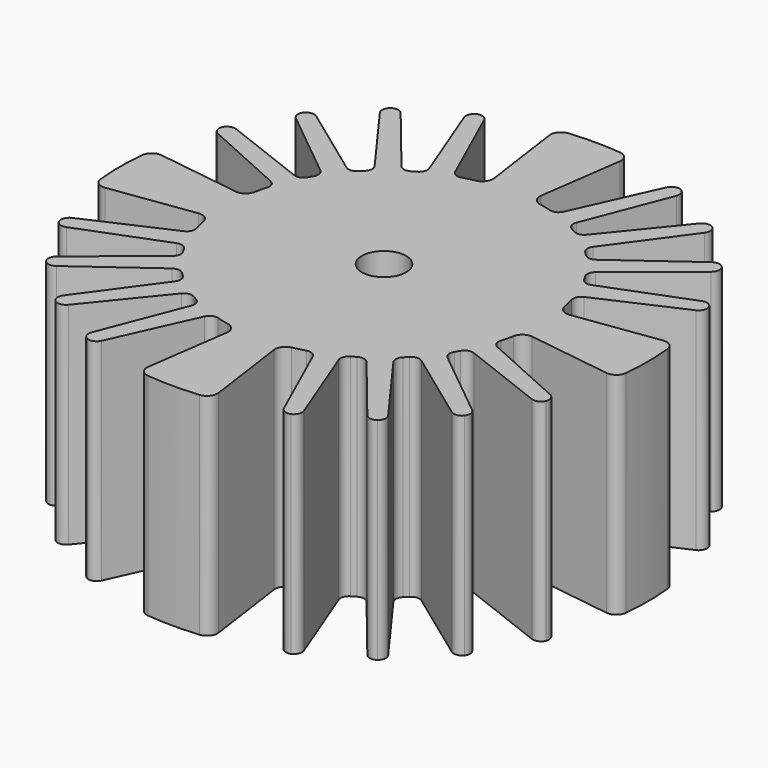
from build123d import *

# Parameters (mm, degrees)
F1_DEPTH        = 20
F2_DEPTH        = 20
F3_R            = 1
F4_DEPTH        = 20
F4_COPIES_COUNT = 4
F4_COPIES_ANGLE = 44.6001
F5_T1_DEPTH     = 20
F5_T3_DEPTH     = 23.9033983658
F6_COUNT        = 4


# Not quite as in the source:
# - a fillet or chamfer that OpenCascade refuses, or shapes differently, is made with other operations: its cross-section is extruded or revolved along the edge and cut away or added
# - a pattern or mirror of a feature is missing from the dataset's text; its kind, count and spacing are read off the source's solid


with BuildPart() as f1:
    # F0 (on Top) → F1 (new body)
    with BuildSketch(Plane.XY):
        with BuildLine():
            ThreePointArc((15, 0), (12.7601203075, 7.8853871013), (6.7094227017, 13.4157984112))
            ThreePointArc((6.7094227017, 13.4157984112), (5.7885906349, 13.8380713418), (4.8413562627, 14.19722753))
            ThreePointArc((4.8413562627, 14.19722753), (3.4800059012, 14.5907353799), (2.0875965144, 14.8540210311))
            ThreePointArc((2.0875965144, 14.8540210311), (0, 15), (-2.0875965144, 14.8540210311))
            ThreePointArc((-2.0875965144, 14.8540210311), (-9.8408854349, -11.3206437033), (15, 0))
        make_face()
    extrude(amount=F1_DEPTH)

    # F0 (on Top) → F2 (join, through all)
    with BuildSketch(Plane.XY):
        with BuildLine():
            ThreePointArc((3.479327524, 24.7567017185), (0, 25), (-3.479327524, 24.7567017185))
            Line((-3.479327524, 24.7567017185), (-2.0875965144, 14.8540210311))
            ThreePointArc((-2.0875965144, 14.8540210311), (0, 15), (2.0875965144, 14.8540210311))
            Line((2.0875965144, 14.8540210311), (3.479327524, 24.7567017185))
        make_face()
    extrude(amount=F2_DEPTH)

    # F3
    f3_edges = [f1.edges().sort_by_distance(p)[0] for p in [
        (-2.087597, 14.854021, 10),
        (-3.479328, 24.756702, 10),
        (3.479328, 24.756702, 10),
        (2.087597, 14.854021, 10),
    ]]
    fillet(f3_edges, radius=F3_R)

    # F0 (on Top) → F4 (join, through all)
    with BuildSketch(Plane.XY):
        with BuildLine():
            Line((6.7094227017, 13.4157984112), (10.335212205, 22.7636418149))
            ThreePointArc((10.335212205, 22.7636418149), (9.6476510581, 23.0634522364), (8.9514050708, 23.3425008784))
            Line((8.9514050708, 23.3425008784), (4.8413562627, 14.19722753))
            ThreePointArc((4.8413562627, 14.19722753), (5.7885906349, 13.8380713418), (6.7094227017, 13.4157984112))
        make_face()
    f4 = extrude(amount=F4_DEPTH)

    # F4_copies: F4 ×4 about axis
    f4_copies_axis = Axis((0, 0, 0), (0, 0, -1))
    for i in range(1, F4_COPIES_COUNT):
        add(f4.rotate(f4_copies_axis, i * F4_COPIES_ANGLE / (F4_COPIES_COUNT - 1)))

    # F5: fillet of radius 0.8 on 16 edges, made by hand

    # F5_s2 → F5_t1 (join)
    with BuildSketch(Plane.XY):
        with BuildLine():
            ThreePointArc((7.3220263558, 13.0915213037), (6.959787066, 13.5188642005), (6.9666753871, 14.0790354293))
            Line((6.9666753871, 14.0790354293), (6.7094227017, 13.4157984112))
            ThreePointArc((6.7094227017, 13.4157984112), (7.0175978493, 13.2571988152), (7.3220263558, 13.0915213037))
        make_face()
        with BuildLine():
            ThreePointArc((4.1803209901, 14.4057251265), (4.7389476864, 14.447861437), (5.1329675358, 14.8460920395))
            Line((5.1329675358, 14.8460920395), (4.8413562627, 14.19722753))
            ThreePointArc((4.8413562627, 14.19722753), (4.5120430988, 14.3052950712), (4.1803209901, 14.4057251265))
        make_face()
        with BuildLine():
            ThreePointArc((13.091534083, 7.3220035068), (13.5188763476, 6.9597634711), (14.0790475884, 6.9666508146))
            Line((14.0790475884, 6.9666508146), (13.4158101213, 6.7093992867))
            ThreePointArc((13.4158101213, 6.7093992867), (13.2572110632, 7.0175747111), (13.091534083, 7.3220035068))
        make_face()
        with BuildLine():
            ThreePointArc((12.850962628, 7.736456523), (12.7483619376, 8.2871945304), (13.0321686521, 8.7701986746))
            Line((13.0321686521, 8.7701986746), (12.47984289, 8.3218700687))
            ThreePointArc((12.47984289, 8.3218700687), (12.6687846419, 8.0313072221), (12.850962628, 7.736456523))
        make_face()
        with BuildLine():
            ThreePointArc((14.4057324225, 4.1802958473), (14.447869708, 4.7389224701), (14.8461009982, 5.1329416245))
            Line((14.8461009982, 5.1329416245), (14.1972359797, 4.8413314838))
            ThreePointArc((14.1972359797, 4.8413314838), (14.3053029462, 4.5120181313), (14.4057324225, 4.1802958473))
        make_face()
        with BuildLine():
            ThreePointArc((11.8203153, 10.3457213754), (11.280662683, 10.1953408334), (10.7746852233, 10.4358113407))
            ThreePointArc((10.7746852233, 10.4358113407), (11.0129238564, 10.1840811138), (11.2452827749, 9.9269136851))
            Line((11.2452827749, 9.9269136851), (11.8203153, 10.3457213754))
        make_face()
        with BuildLine():
            ThreePointArc((10.435830146, 10.7746670094), (10.1953605219, 11.2806448887), (10.3457420057, 11.8202972433))
            Line((10.3457420057, 11.8202972433), (9.9269333118, 11.2452654492))
            ThreePointArc((9.9269333118, 11.2452654492), (10.184100335, 11.0129060818), (10.435830146, 10.7746670094))
        make_face()
        with BuildLine():
            ThreePointArc((8.77022142, 13.0321533452), (8.2872167805, 12.7483474737), (7.7364789522, 12.8509491254))
            ThreePointArc((7.7364789522, 12.8509491254), (8.0313293333, 12.6687706246), (8.3218918501, 12.4798283656))
            Line((8.3218918501, 12.4798283656), (8.77022142, 13.0321533452))
        make_face()
    extrude(amount=F5_T1_DEPTH)

    # F5_s4 → F5_t3 (cut)
    with BuildSketch(Plane.XY.offset(-1.9516991829)):
        with BuildLine():
            ThreePointArc((10.0574529871, 22.0475357998), (10.0475329409, 22.6505133096), (9.6194152336, 23.0752432395))
            ThreePointArc((9.6194152336, 23.0752432395), (9.9785300979, 22.9222367383), (10.335212205, 22.7636418149))
            Line((10.335212205, 22.7636418149), (10.0574529871, 22.0475357998))
        make_face()
        with BuildLine():
            ThreePointArc((9.6758724299, 23.0516266828), (9.072849502, 23.0582322241), (8.6365484192, 22.641913056))
            Line((8.6365484192, 22.641913056), (8.9514050708, 23.3425008784))
            ThreePointArc((8.9514050708, 23.3425008784), (9.3147742174, 23.1998918377), (9.6758724299, 23.0516266828))
        make_face()
        with BuildLine():
            ThreePointArc((19.6681191788, 14.1566692198), (19.9585608877, 14.68518024), (19.7974592245, 15.2663226827))
            ThreePointArc((19.7974592245, 15.2663226827), (20.0334080786, 14.9553522445), (20.2644728046, 14.6407357039))
            Line((20.2644728046, 14.6407357039), (19.6681191788, 14.1566692198))
        make_face()
        with BuildLine():
            ThreePointArc((19.8347704257, 15.2178146315), (19.3144160793, 15.5226287369), (18.729077574, 15.3775111335))
            Line((18.729077574, 15.3775111335), (19.3499480002, 15.829703484))
            ThreePointArc((19.3499480002, 15.829703484), (19.5947478045, 15.5256516282), (19.8347704257, 15.2178146315))
        make_face()
        with BuildLine():
            ThreePointArc((15.3775438218, 18.7290507351), (15.5226624469, 19.3143889872), (15.2178492497, 19.8347438656))
            ThreePointArc((15.2178492497, 19.8347438656), (15.5256858274, 19.5947207071), (15.829737256, 19.3499203721))
            Line((15.829737256, 19.3499203721), (15.3775438218, 18.7290507351))
        make_face()
        with BuildLine():
            ThreePointArc((15.2663572358, 19.7974325797), (14.6852150742, 19.9585352572), (14.1567035471, 19.6680944707))
            Line((14.1567035471, 19.6680944707), (14.640771072, 20.2644472517))
            ThreePointArc((14.640771072, 20.2644472517), (14.9553872093, 20.0333819766), (15.2663572358, 19.7974325797))
        make_face()
        with BuildLine():
            ThreePointArc((23.0752600286, 9.6193749597), (22.6505308459, 10.0474934083), (22.0475533533, 10.0574145068))
            Line((22.0475533533, 10.0574145068), (22.7636598532, 10.3351724749))
            ThreePointArc((22.7636598532, 10.3351724749), (22.9222541541, 9.978490091), (23.0752600286, 9.6193749597))
        make_face()
        with BuildLine():
            ThreePointArc((22.6419281296, 8.6365089016), (23.0582480592, 9.0728092578), (23.0516435703, 9.6758321972))
            ThreePointArc((23.0516435703, 9.6758321972), (23.199908095, 9.3147337259), (23.3425165015, 8.9513643304))
            Line((23.3425165015, 8.9513643304), (22.6419281296, 8.6365089016))
        make_face()
    extrude(amount=F5_T3_DEPTH, mode=Mode.SUBTRACT)


with BuildPart() as f6_1:
    # F6: instance of F1
    add(f1.part.rotate(Axis((0, 0, 0), (0, 0, -1)), 1 * 360 / F6_COUNT))


with BuildPart() as f6_2:
    # F6: instance of F1
    add(f1.part.rotate(Axis((0, 0, 0), (0, 0, -1)), 2 * 360 / F6_COUNT))


with BuildPart() as f6_3:
    # F6: instance of F1
    add(f1.part.rotate(Axis((0, 0, 0), (0, 0, -1)), 3 * 360 / F6_COUNT))


with BuildPart() as f1_1:
    add(f1.part)

    # F7: union F6_1, F6_3, F6_2
    add(f6_1.part)
    add(f6_3.part)
    add(f6_2.part)

    # F8 (on Front) → F9 (revolve, cut)
    with BuildSketch(Plane.XZ):
        Polygon((0, 20), (0, 0), (1, 0), (1, 17), (2.1, 17), (2.1, 20), align=None)
    revolve(axis=Axis((0, 0, 11.9276111946), (0, 0, 1)), mode=Mode.SUBTRACT)


solid = f1_1.part
